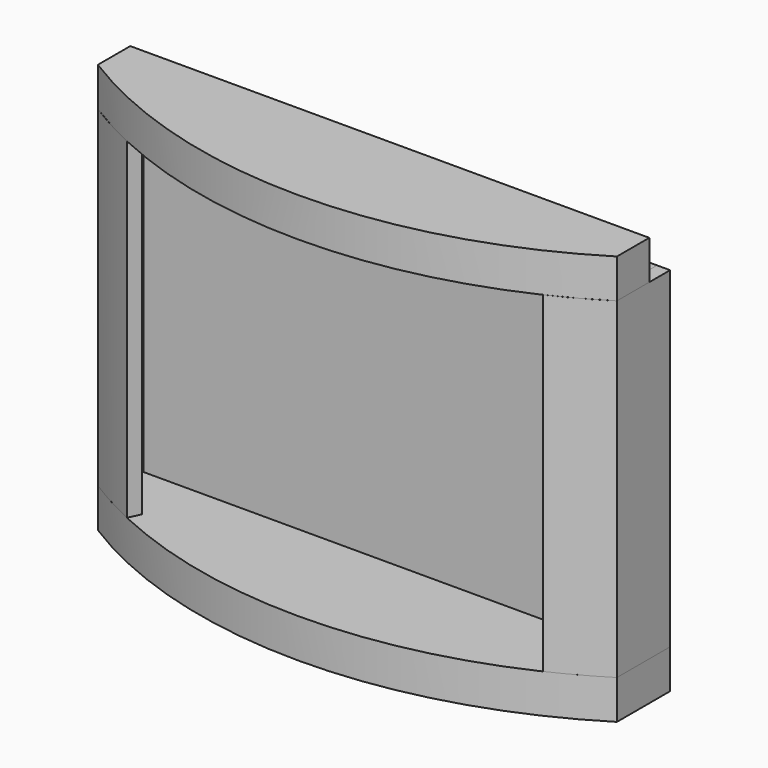
from build123d import *

# Parameters (mm, degrees)
F1_DEPTH = 33
F4_DEPTH = 33
F5_DEPTH = 22
F7_DEPTH = 280
F8_W     = 416.265957
F8_H     = 22
F9_DEPTH = 280


# Not quite as in the source:
# - ends of sketch curves that miss each other by under 0.0002 mm in the source are joined


with BuildPart() as f1:
    # F0 (on Top) → F1 (new body)
    with BuildSketch(Plane.XY):
        with BuildLine():
            Line((219.132978, 48.5), (-219.132979, 48.5))
            Line((-219.132979, 48.5), (-219.132979, 14.349509))
            ThreePointArc((-219.132979, 14.349509), (-4.24e-07, -48.499999), (219.1329780871, 14.3495088607))
            Line((219.1329780871, 14.3495088607), (219.132978, 48.5))
        make_face()
    extrude(amount=F1_DEPTH)


with BuildPart() as f4:
    # F3 (on offset) → F4 (new body)
    with BuildSketch(Plane(origin=(0, 0, -280), x_dir=(1, 0, 0), z_dir=(0, 0, -1))):
        with BuildLine():
            Line((-219.132979, -14.349509), (-219.132979, -48.5))
            Line((-219.132979, -48.5), (219.132978, -48.5))
            Line((219.132978, -48.5), (219.132978, -14.3495088607))
            ThreePointArc((219.132978, -14.3495088607), (-4.24e-07, 48.499999), (-219.132979, -14.349509))
        make_face()
    extrude(amount=F4_DEPTH)

    # F5 (add): a face of the model
    f5_faces = [f4.faces().sort_by_distance(p)[0] for p in [
        (-5e-07, 48.5, -296.5),
    ]]
    extrude(f5_faces, amount=F5_DEPTH)


with BuildPart() as f7:
    # F6 (on face) → F7 (new body)
    with BuildSketch(Plane.XY.offset(-280)):
        with BuildLine():
            ThreePointArc((175.6739587965, -9.3212637837), (197.7579472725, 1.8633071047), (219.1329780245, 14.3495088216))
            Line((219.132978, 14.3495088607), (219.132978, 70.5))
            Line((219.132978, 70.5), (208.132978, 70.5))
            Line((208.132978, 70.5), (208.132978, 20.5000005459))
            ThreePointArc((208.132978, 20.5000005459), (189.82648619, 10.0821389395), (170.9999998518, 0.6363517834))
            Line((170.9999998518, 0.6363517834), (175.6739587965, -9.3212637837))
        make_face()
    extrude(amount=F7_DEPTH)


with BuildPart() as f7b:
    # F6 (on face) → F7, piece 2 (new body)
    with BuildSketch(Plane.XY.offset(-280)):
        with BuildLine():
            Line((-208.132979, 70.5), (-219.132979, 70.5))
            Line((-219.132979, 70.5), (-219.132979, 14.349509))
            ThreePointArc((-219.132979, 14.349509), (-197.7579478249, 1.8633074056), (-175.673959101, -9.3212636408))
            Line((-175.673959101, -9.3212636408), (-171.0000001482, 0.6363519225))
            ThreePointArc((-171.0000001482, 0.6363519225), (-189.8264868494, 10.0821392923), (-208.132979, 20.5000011501))
            Line((-208.132979, 20.5000011501), (-208.132979, 70.5))
        make_face()
    extrude(amount=F7_DEPTH)


with BuildPart() as f9:
    # F8 (on face) → F9 (new body)
    with BuildSketch(Plane.XY.offset(-280)):
        with Locations((-5e-07, 59.5)):
            Rectangle(F8_W, F8_H)
    extrude(amount=F9_DEPTH)


solid = Compound([f1.part, f4.part, f7.part, f7b.part, f9.part])
